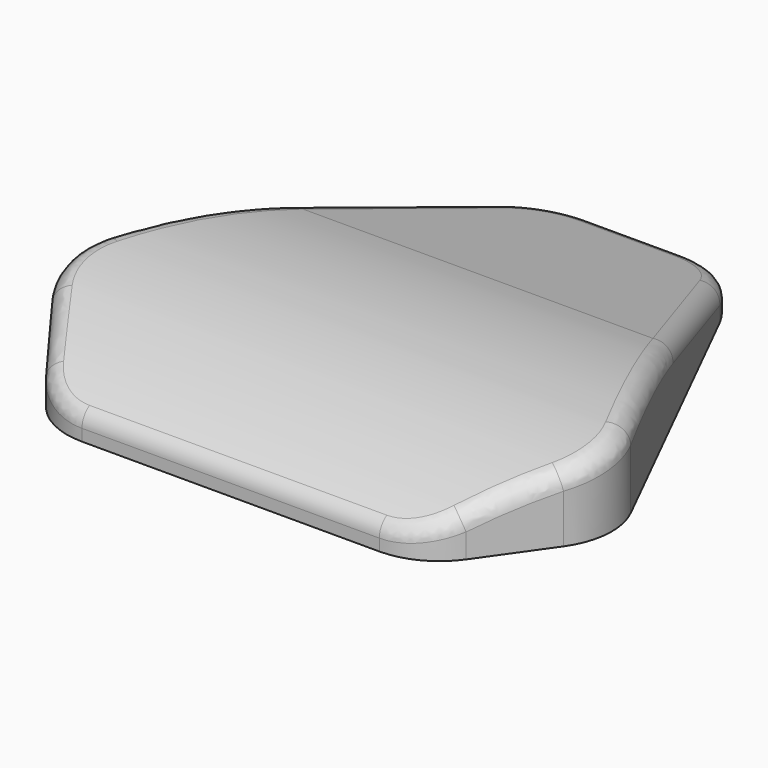
from build123d import *

# Parameters (mm, degrees)
F1_DEPTH    = 7.62
F2_SIZE2    = 6.096
F2_SIZE     = 9.017
F3_T1_DEPTH = 145.1738679331
F4_R        = 5.08
F5_T1_DEPTH = 97.646763874
F6_R        = 1.27


# Not quite as in the source:
# - a fillet or chamfer that OpenCascade refuses, or shapes differently, is made with other operations: its cross-section is extruded or revolved along the edge and cut away or added


with BuildPart() as f1:
    # F0 (on Top) → F1 (new body)
    with BuildSketch(Plane.XY):
        Polygon((-19.05, -8.4781497717), (-12.7, -17.4958198279), (12.7, -17.4958198279), (19.05, -8.4781497717), (6.35, 17.0205775648), (-6.35, 17.0205775648), align=None)
    extrude(amount=F1_DEPTH)

    # F2
    f2_edges = [f1.edges().sort_by_distance(p)[0] for p in [
        (0, -17.49582, 7.62),
    ]]
    f2_side = f1.faces().sort_by_distance((0, -2.400647, 7.62))[0]
    chamfer(f2_edges, length=F2_SIZE, length2=F2_SIZE2, reference=f2_side)

    # F3: chamfer of 25.5016 x 6.096 on 1 edges, made by hand

    # F3_s2 → F3_t1 (cut)
    with BuildSketch(Plane.YZ.offset(-72.5869339665)):
        Polygon((-8.4810224352, 7.62), (17.0205775648, 1.524), (17.0205775648, 7.62), align=None)
    extrude(amount=F3_T1_DEPTH, mode=Mode.SUBTRACT)

    # F4
    f4_edges = [f1.edges().sort_by_distance(p)[0] for p in [
        (19.05, -8.47815, 3.809657),
        (12.7, -17.49582, 0.762),
        (-12.7, -17.49582, 0.762),
        (-19.05, -8.47815, 3.809657),
        (6.35, 17.020578, 0.762),
        (-6.35, 17.020578, 0.762),
    ]]
    fillet(f4_edges, radius=F4_R)

    # F5: fillet of radius 27.94 on 1 edges, made by hand

    # F5_s2 → F5_t1 (cut)
    with BuildSketch(Plane.YZ.offset(-48.823381937)):
        with BuildLine():
            ThreePointArc((-17.4958198279, 1.524), (-7.3528274709, 5.2076739368), (3.4295965216, 4.77284009))
            Line((3.4295965216, 4.77284009), (-8.4793951963, 7.6196110186))
            Line((-8.4793951963, 7.6196110186), (-17.4958198279, 1.524))
        make_face()
    extrude(amount=F5_T1_DEPTH, mode=Mode.SUBTRACT)

    # F6
    f6_edges = [f1.edges().sort_by_distance(p)[0] for p in [
        (0, -17.49582, 1.524),
        (-15.736261, -13.184009, 3.642167),
        (-18.210711, -8.494691, 5.006042),
        (-12.356582, -16.949127, 1.845308),
        (-15.396033, -1.141811, 5.472098),
        (15.396033, -1.141811, 5.472098),
        (18.210711, -8.494691, 5.006042),
        (15.736261, -13.184009, 3.642167),
        (12.356317, -16.949258, 1.845234),
        (-10.435665, 8.817487, 3.484898),
        (-5.879006, 16.259813, 1.705856),
        (0, 17.020578, 1.524),
        (5.879006, 16.259813, 1.705856),
        (10.435665, 8.817487, 3.484898),
    ]]
    fillet(f6_edges, radius=F6_R)


solid = f1.part
